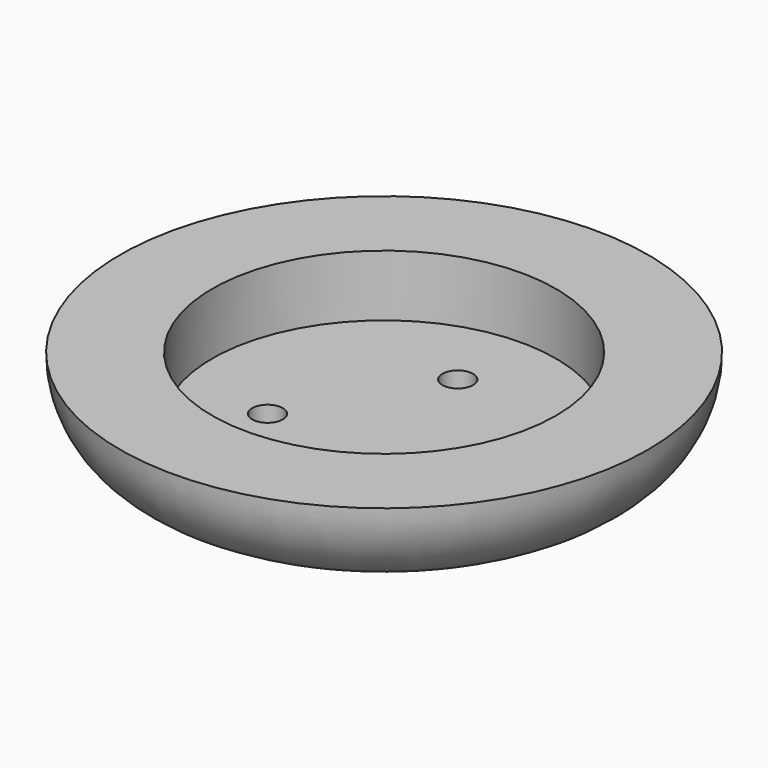
from build123d import *

# Parameters (mm, degrees)
F2_R           = 14.99999
F4_D           = 5
F4_CBORE_D     = 8
F4_CBORE_DEPTH = 2


# Not quite as in the source:
# - a fillet or chamfer is up to 0.001 mm smaller than in the source, because OpenCascade refuses the exact size


with BuildPart() as f1:
    # F0 (on Front) → F1 (revolve)
    with BuildSketch(Plane.XZ):
        Polygon((28, -25), (0, -25), (0, -30), (43, -30), (43, -15), (28, -15), align=None)
    revolve(axis=Axis((0, 0, -27.5), (0, 0, 1)))

    # F2 (radius 15 in the source; OpenCascade refuses exactly that, so slightly less here)
    f2_edges = [f1.edges().sort_by_distance(p)[0] for p in [
        (-43, 0, -30),
    ]]
    fillet(f2_edges, radius=F2_R)

    # F4 (through all)
    with Locations(Plane(origin=(0, 0, -30), x_dir=(1, 0, 0), z_dir=(0, 0, -1))):
        with Locations((-12.9903810568, 7.5), (12.9903810568, 7.5), (0, -15)):
            CounterBoreHole(F4_D / 2, F4_CBORE_D / 2, F4_CBORE_DEPTH)


solid = f1.part
